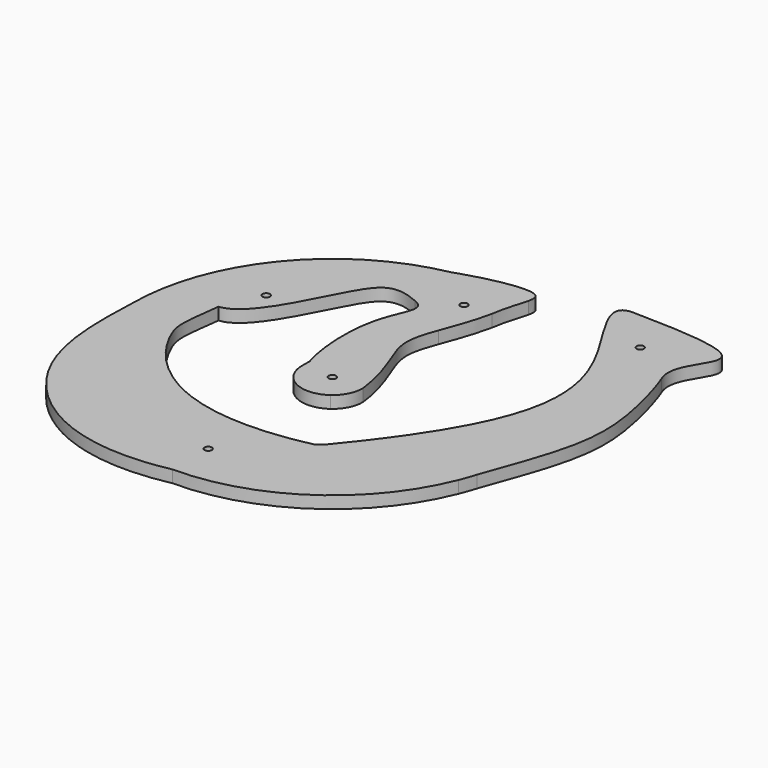
from build123d import *

# Parameters (mm, degrees)
F0_W     = 200
F0_H     = 200
F1_DEPTH = 5
F2_R     = 1.5
F3_DEPTH = 5.001
F4_W     = 200
F4_H     = 200
F5_DEPTH = 5.001


with BuildPart() as f1:
    # F0 (on Top) → F1 (new body)
    with BuildSketch(Plane.XY):
        Rectangle(F0_W, F0_H)
    extrude(amount=F1_DEPTH)

    # F2 (on face) → F3 (cut, through all)
    with BuildSketch(Plane.XY.offset(5)):
        Circle(F2_R)
        with Locations((0, -63.662)):
            Circle(F2_R)
        with Locations((64.1583176089, 77.5462182691)):
            Circle(F2_R)
        with Locations((-51.9230208324, 31.0114389966)):
            Circle(F2_R)
        with Locations((1.6717778053, 65.3690844774)):
            Circle(F2_R)
    extrude(amount=-F3_DEPTH, mode=Mode.SUBTRACT)

    # F4 (on face) → F5 (cut, through all)
    with BuildSketch(Plane.XY.offset(5)):
        Rectangle(F4_W, F4_H)
        with BuildLine():
            ThreePointArc((-82, 0), (-77.2870838173, 27.3990268992), (-63.690081097, 51.6485582554))
            ThreePointArc((-63.690081097, 51.6485582554), (-42.2483285841, 70.2785794666), (-15.7371131629, 80.4757309336))
            add(Edge.make_bspline(
                [(-12.5, 81.5484393368), (-13.565916229, 81.2087498873), (-14.6459371087, 80.8510464166), (-15.7371131629, 80.4757309336)],
                knots=[0.6055452202, 0.6055452202, 0.6055452202, 0.6055452202, 0.6293477845, 0.6293477845, 0.6293477845, 0.6293477845], degree=3))
            Line((-12.5, 81.5484393368), (-12.5, 82))
            ThreePointArc((-12.5, 82), (-2.0170867918, 94.336180968), (11.8490177399, 85.9813036306))
            add(Edge.make_bspline(
                [(16.0253920965, 80.4188212308), (16.5650357956, 82.8751284088), (16.3522810864, 85.1091068393), (12.9758843421, 85.8767877596), (11.8490177399, 85.9813036306)],
                knots=[0.1836933529, 0.1836933529, 0.1836933529, 0.1836933529, 0.3224690729, 0.3745974074, 0.3745974074, 0.3745974074, 0.3745974074], degree=3))
            ThreePointArc((16.0253920965, 80.4188212308), (40.6644445944, 71.2067619389), (61.1188515162, 54.6670466492))
            add(Edge.make_bspline(
                [(61.1188515162, 54.6670466492), (59.6886774699, 58.4839230093), (50.943301884, 76.7103239151), (34.6142351627, 96.1605012417), (48.7091802061, 95.0762778521)],
                knots=[0.5656722023, 0.5656722023, 0.5656722023, 0.5656722023, 0.6560716463, 1, 1, 1, 1], degree=3))
            add(Edge.make_bspline(
                [(48.7091802061, 95.0762778521), (117.6007725298, 94.2181646824), (75.5295977616, 82.3686383673), (82.9158574343, 65.1235729456)],
                knots=[0, 0, 0, 0, 45.4671452613, 45.4671452613, 45.4671452613, 45.4671452613], degree=3))
            add(Edge.make_bspline(
                [(78.4521397815, -23.8592071056), (86.8162837408, -0.2995062418), (96.8687794415, 24.2860117165), (84.4595443335, 61.4847043894), (82.9158574343, 65.1235729456)],
                knots=[0.0470183009, 0.0470183009, 0.0470183009, 0.0470183009, 0.5706356913, 1, 1, 1, 1], degree=3))
            ThreePointArc((78.4521397815, -23.8592071056), (77.3630287515, -27.1838515004), (76.1330969529, -30.4590142381))
            ThreePointArc((76.1330969529, -30.4590142381), (45.9693421341, -67.9030160137), (0, -82))
            add(Edge.make_bspline(
                [(-82, 0), (-82.9754887272, -20.7067543445), (-82.1344867438, -60.3498402786), (-36.9418002665, -89.5115286112), (0, -82)],
                knots=[0, 0, 0, 0, 0.4580463953, 1, 1, 1, 1], degree=3))
        make_face(mode=Mode.SUBTRACT)
        with BuildLine():
            Line((-12.5, 43.2061646239), (-12.5, 45.3072841826))
            ThreePointArc((-12.5, 45.3072841826), (-46.3706934869, 7.665427943), (-26.4158389737, -38.8742003302))
            add(Edge.make_bspline(
                [(-26.4158389737, -38.8742003302), (-14.0577632879, -43.3636988671), (2.4642567557, -44.9462907372), (24.3826498161, -40.1806718205)],
                knots=[0.7302795759, 0.7302795759, 0.7302795759, 0.7302795759, 0.982187731, 0.982187731, 0.982187731, 0.982187731], degree=3))
            ThreePointArc((24.3826498161, -40.1806718205), (25.742641555, -39.3232298492), (27.0725114402, -38.4197751727))
            add(Edge.make_bspline(
                [(27.0725114402, -38.4197751727), (33.7652480292, -30.3154217605), (39.4471667486, -22.864238901), (44.2099042851, -15.952566035)],
                knots=[0, 0, 0, 0, 0.1032371867, 0.1032371867, 0.1032371867, 0.1032371867], degree=3))
            ThreePointArc((44.2099042851, -15.952566035), (46.2972218465, -8.0973606379), (47, 0))
            ThreePointArc((47, 0), (37.3931811966, 28.4736720498), (12.5, 45.3072841826))
            Line((12.5, 45.3072841826), (12.5, 0))
            ThreePointArc((12.5, 0), (11.1416208558, -5.6669466827), (7.3617144473, -10.1022354158))
            ThreePointArc((7.3617144473, -10.1022354158), (-5.6669466827, -11.1416208558), (-12.5, 0))
            Line((-12.5, 0), (-12.5, 4.025513493))
            add(Edge.make_bspline(
                [(-12.5, 43.2061646239), (-13.0556807874, 41.6106183041), (-16.1819671512, 31.276628776), (-15.7702054334, 14.6129505283), (-12.5, 4.025513493)],
                knots=[0.3190961461, 0.3190961461, 0.3190961461, 0.3190961461, 0.3816066867, 0.6867466968, 0.6867466968, 0.6867466968, 0.6867466968], degree=3))
        make_face()
        with BuildLine():
            ThreePointArc((61.1188515162, 54.6670466492), (40.6644445944, 71.2067619389), (16.0253920965, 80.4188212308))
            add(Edge.make_bspline(
                [(12.5, 66.1564320326), (13.3802789518, 72.4577917019), (15.3110815492, 77.1674794144), (16.0253920965, 80.4188212308)],
                knots=[0, 0, 0, 0, 0.1836933529, 0.1836933529, 0.1836933529, 0.1836933529], degree=3))
            Line((12.5, 66.1564320326), (12.5, 45.3072841826))
            ThreePointArc((12.5, 45.3072841826), (37.3931811966, 28.4736720498), (47, 0))
            ThreePointArc((47, 0), (46.2972218465, -8.0973606379), (44.2099042851, -15.952566035))
            add(Edge.make_bspline(
                [(44.2099042851, -15.952566035), (65.5438506797, 15.0072039057), (68.4348540043, 35.1419566642), (61.1188515162, 54.6670466492)],
                knots=[0.1032371867, 0.1032371867, 0.1032371867, 0.1032371867, 0.5656722023, 0.5656722023, 0.5656722023, 0.5656722023], degree=3))
        make_face()
        with BuildLine():
            Line((-12.5, 45.3072841826), (-12.5, 57.8710343872))
            add(Edge.make_bspline(
                [(-12.5, 57.8710343872), (-23.5213679573, 62.6746186598), (-32.8095018381, 54.3189817446), (-48.0139010469, 16.1354373957), (-58.9577592909, 15.3648024425)],
                knots=[0, 0, 0, 0, 0.4048381089, 1, 1, 1, 1], degree=3))
            add(Edge.make_bspline(
                [(-58.9577592909, 15.3648024425), (-60.8916521811, 0), (-62.6803618933, -6.109964317), (-45.3110909102, -32.009846358), (-26.4158389737, -38.8742003302)],
                knots=[0, 0, 0, 0, 0.345117017, 0.7302795759, 0.7302795759, 0.7302795759, 0.7302795759], degree=3))
            ThreePointArc((-26.4158389737, -38.8742003302), (-46.3706934869, 7.665427943), (-12.5, 45.3072841826))
        make_face()
        with BuildLine():
            ThreePointArc((12.5, 45.3072841826), (9.4442668294, 46.0413490686), (6.3463086948, 46.5695648031))
            add(Edge.make_bspline(
                [(12.5, 0), (10.5419723461, 16.7892477372), (0.3817668008, 28.6317596489), (4.5429672006, 41.6113561468), (6.3463086948, 46.5695648031)],
                knots=[0, 0, 0, 0, 0.5018890592, 0.7412506552, 0.7412506552, 0.7412506552, 0.7412506552], degree=3))
            Line((12.5, 0), (12.5, 45.3072841826))
        make_face()
        with BuildLine():
            Line((-12.5, 82), (-12.5, 81.5484393368))
            add(Edge.make_bspline(
                [(11.8490177399, 85.9813036306), (6.8565816762, 86.444347617), (-2.1577940468, 84.8443252147), (-12.5, 81.5484393368)],
                knots=[0.3745974074, 0.3745974074, 0.3745974074, 0.3745974074, 0.6055452202, 0.6055452202, 0.6055452202, 0.6055452202], degree=3))
            ThreePointArc((11.8490177399, 85.9813036306), (-2.0170867918, 94.336180968), (-12.5, 82))
        make_face()
        with BuildLine():
            Line((12.5, 45.3072841826), (12.5, 66.1564320326))
            add(Edge.make_bspline(
                [(6.3463086948, 46.5695648031), (8.295716779, 51.9293771678), (10.7822211501, 58.1853447453), (12.5, 66.1564320326)],
                knots=[0.7412506552, 0.7412506552, 0.7412506552, 0.7412506552, 1, 1, 1, 1], degree=3))
            ThreePointArc((6.3463086948, 46.5695648031), (9.4442668294, 46.0413490686), (12.5, 45.3072841826))
        make_face()
        with BuildLine():
            add(Edge.make_bspline(
                [(-12.5, 57.8710343872), (-6.8313528953, 55.5466772944), (-9.0656623287, 52.1282588916), (-11.636455957, 45.5367202679)],
                knots=[0, 0, 0, 0, 0.2870336806, 0.2870336806, 0.2870336806, 0.2870336806], degree=3))
            Line((-12.5, 57.8710343872), (-12.5, 45.3072841826))
            ThreePointArc((-12.5, 45.3072841826), (-12.068773209, 45.424054346), (-11.636455957, 45.5367202679))
        make_face()
        with BuildLine():
            ThreePointArc((-11.636455957, 45.5367202679), (-12.068773209, 45.424054346), (-12.5, 45.3072841826))
            Line((-12.5, 45.3072841826), (-12.5, 43.2061646239))
            add(Edge.make_bspline(
                [(-11.636455957, 45.5367202679), (-11.9236208006, 44.8004269549), (-12.2149841308, 44.0245409859), (-12.5, 43.2061646239)],
                knots=[0.2870336806, 0.2870336806, 0.2870336806, 0.2870336806, 0.3190961461, 0.3190961461, 0.3190961461, 0.3190961461], degree=3))
        make_face()
    extrude(amount=-F5_DEPTH, mode=Mode.SUBTRACT)


solid = f1.part
